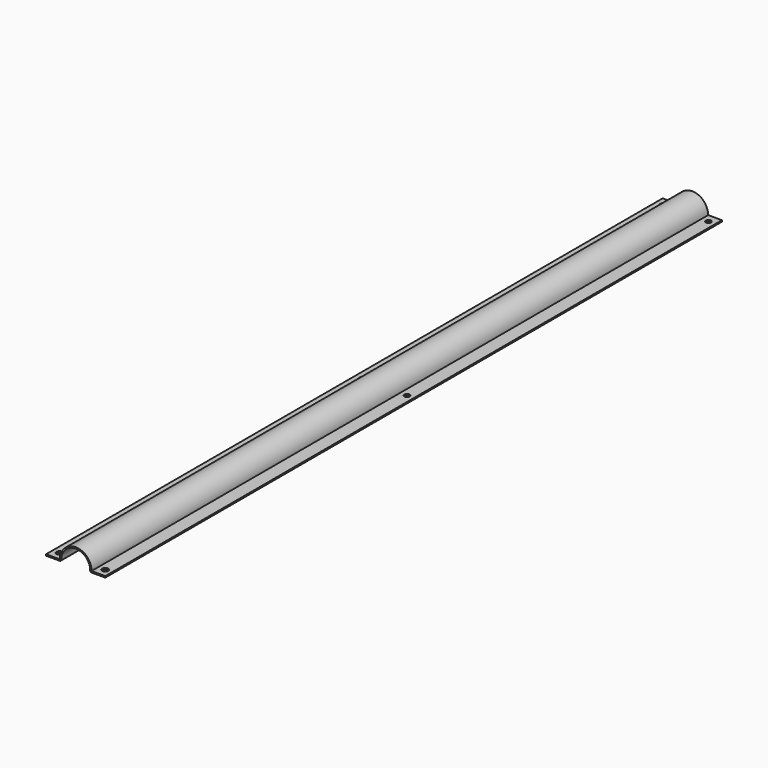
from build123d import *

# Parameters (mm, degrees)
F1_DEPTH = 559.5
F2_R     = 1.9
F2_R_2   = 2.2432813823
F3_DEPTH = 1


# Not quite as in the source:
# - a pattern or mirror of a feature is missing from the dataset's text; its kind, count and spacing are read off the source's solid
# - a feature names something its author has since deleted; it is built from what else it names


with BuildPart() as f1:
    # F0 (on Front) → F1 (new body)
    with BuildSketch(Plane.XZ):
        with BuildLine():
            Line((-21.5, 0), (-21.5, -1))
            Line((-21.5, -1), (-11.5475115549, -1))
            ThreePointArc((-11.5475115549, -1), (-10.8404047737, -0.7071067812), (-10.5475115549, 0))
            ThreePointArc((-10.5475115549, 0), (0, 10.5475115549), (10.5475115549, 0))
            ThreePointArc((10.5475115549, 0), (10.8404047737, -0.7071067812), (11.5475115549, -1))
            Line((11.5475115549, -1), (21.5, -1))
            Line((21.5, -1), (21.5, 0))
            Line((21.5, 0), (11.5, 0))
            ThreePointArc((11.5, 0), (0, 11.5), (-11.5, 0))
            Line((-11.5, 0), (-21.5, 0))
        make_face()
    extrude(amount=F1_DEPTH)

    # F2 (on face) → F3 (cut, through all)
    with BuildSketch(Plane.XY):
        with Locations((16.5, -279.50005)):
            Circle(F2_R)
        with Locations((16.5, -6)):
            Circle(F2_R)
        with Locations((16.5236079696, -553.5000464449)):
            Circle(F2_R_2)
    f3 = extrude(amount=-F3_DEPTH, mode=Mode.SUBTRACT)

    # F3_copies: F3 across plane
    add(f3.mirror(Plane(origin=(0, 0, 0), x_dir=(0, 0, -1), z_dir=(-1, 0, 0))), mode=Mode.SUBTRACT)


solid = f1.part
